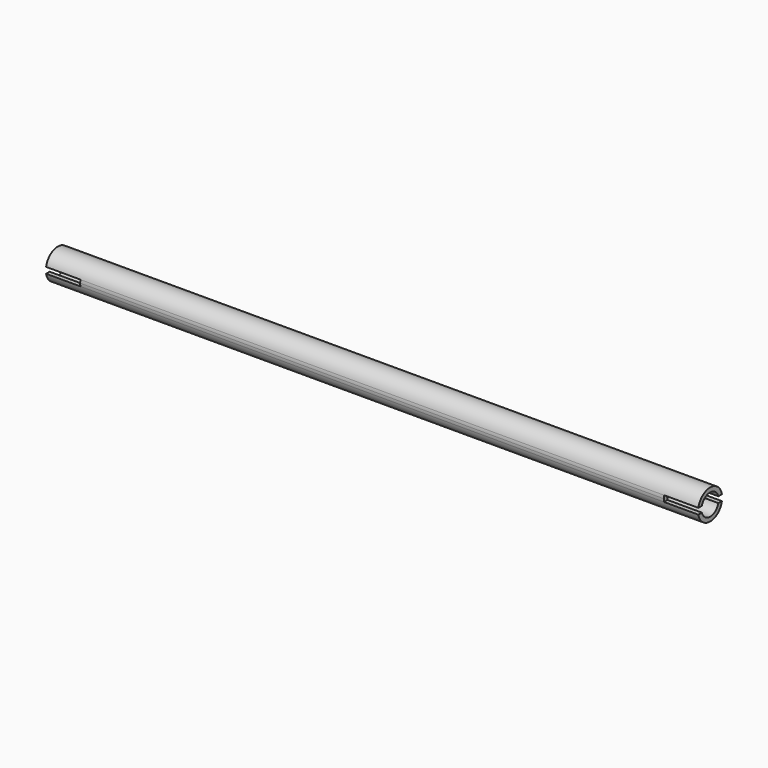
from build123d import *
from build123d import SkipClean  # not in build123d's __all__

# Parameters (mm, degrees)
F0_R          = 11.1125
F0_R_2        = 7.9375
F1_DEPTH      = 241.2365
F1_DEPTH_BACK = 241.2365
F3_DEPTH      = 482.474
F4_DEPTH      = 457.073
F5_DEPTH      = 25.4


with BuildPart() as f1:
    # F0 (on Right) → F1 (new body, two sides)
    with BuildSketch(Plane.YZ) as f1_sk:
        Circle(F0_R)
        Circle(F0_R_2, mode=Mode.SUBTRACT)
    extrude(amount=F1_DEPTH)
    extrude(f1_sk.sketch, amount=-F1_DEPTH_BACK)

    # F2 (on face) → F3 (cut, through all)
    with BuildSketch(Plane.YZ.offset(241.2365)):
        with BuildLine():
            Line((-7.62, 2.2225), (-10.8879819067, 2.2225))
            ThreePointArc((-10.8879819067, 2.2225), (-11.0562280003, 1.1169058403), (-11.1125, 0))
            ThreePointArc((-11.1125, 0), (-11.0562280003, -1.1169058403), (-10.8879819067, -2.2225))
            Line((-10.8879819067, -2.2225), (-7.62, -2.2225))
            ThreePointArc((-7.62, -2.2225), (-7.9375, 0), (-7.62, 2.2225))
        make_face()
        with BuildLine():
            ThreePointArc((11.1125, 0), (11.0562280003, 1.1169058403), (10.8879819067, 2.2225))
            Line((10.8879819067, 2.2225), (7.62, 2.2225))
            ThreePointArc((7.62, 2.2225), (7.8577241059, 1.1225320151), (7.9375, 0))
            ThreePointArc((7.9375, 0), (7.8577241059, -1.1225320151), (7.62, -2.2225))
            Line((7.62, -2.2225), (10.8879819067, -2.2225))
            ThreePointArc((10.8879819067, -2.2225), (11.0562280003, -1.1169058403), (11.1125, 0))
        make_face()
    extrude(amount=-F3_DEPTH, mode=Mode.SUBTRACT)

    # F2 (on face) → F4 (join)
    with BuildSketch(Plane.YZ.offset(241.2365)):
        with BuildLine():
            Line((-7.62, 2.2225), (-10.8879819067, 2.2225))
            ThreePointArc((-10.8879819067, 2.2225), (-11.0562280003, 1.1169058403), (-11.1125, 0))
            ThreePointArc((-11.1125, 0), (-11.0562280003, -1.1169058403), (-10.8879819067, -2.2225))
            Line((-10.8879819067, -2.2225), (-7.62, -2.2225))
            ThreePointArc((-7.62, -2.2225), (-7.9375, 0), (-7.62, 2.2225))
        make_face()
        with BuildLine():
            ThreePointArc((11.1125, 0), (11.0562280003, 1.1169058403), (10.8879819067, 2.2225))
            Line((10.8879819067, 2.2225), (7.62, 2.2225))
            ThreePointArc((7.62, 2.2225), (7.8577241059, 1.1225320151), (7.9375, 0))
            ThreePointArc((7.9375, 0), (7.8577241059, -1.1225320151), (7.62, -2.2225))
            Line((7.62, -2.2225), (10.8879819067, -2.2225))
            ThreePointArc((10.8879819067, -2.2225), (11.0562280003, -1.1169058403), (11.1125, 0))
        make_face()
    with SkipClean():  # cleaning this boolean's faces spoils the solid; the shape is the same uncleaned
        extrude(amount=-F4_DEPTH)

    # F2 (on face) → F5 (cut)
    with BuildSketch(Plane.YZ.offset(241.2365)):
        with BuildLine():
            Line((-7.62, 2.2225), (-10.8879819067, 2.2225))
            ThreePointArc((-10.8879819067, 2.2225), (-11.0562280003, 1.1169058403), (-11.1125, 0))
            ThreePointArc((-11.1125, 0), (-11.0562280003, -1.1169058403), (-10.8879819067, -2.2225))
            Line((-10.8879819067, -2.2225), (-7.62, -2.2225))
            ThreePointArc((-7.62, -2.2225), (-7.9375, 0), (-7.62, 2.2225))
        make_face()
        with BuildLine():
            ThreePointArc((11.1125, 0), (11.0562280003, 1.1169058403), (10.8879819067, 2.2225))
            Line((10.8879819067, 2.2225), (7.62, 2.2225))
            ThreePointArc((7.62, 2.2225), (7.8577241059, 1.1225320151), (7.9375, 0))
            ThreePointArc((7.9375, 0), (7.8577241059, -1.1225320151), (7.62, -2.2225))
            Line((7.62, -2.2225), (10.8879819067, -2.2225))
            ThreePointArc((10.8879819067, -2.2225), (11.0562280003, -1.1169058403), (11.1125, 0))
        make_face()
    with SkipClean():  # cleaning this boolean's faces spoils the solid; the shape is the same uncleaned
        extrude(amount=-F5_DEPTH, mode=Mode.SUBTRACT)


solid = f1.part
